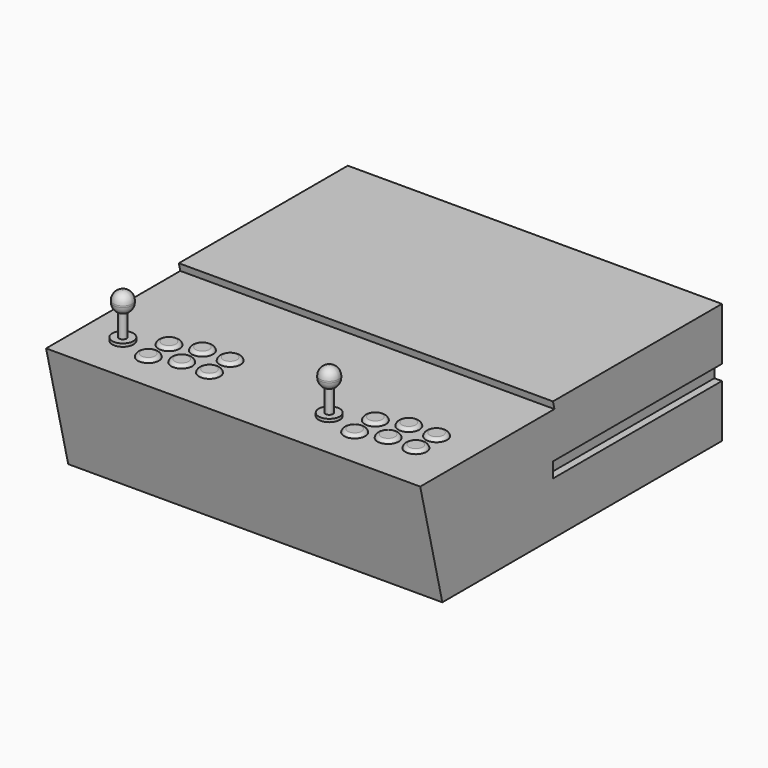
from build123d import *

# Parameters (mm, degrees)
F0_W      = 500
F0_H      = 150
F1_DEPTH  = 500
F3_DEPTH  = 546
F4_W      = 500
F4_H      = 280
F5_DEPTH  = 10
F6_DEPTH  = 2
F7_DEPTH  = 2
F8_W      = 280
F8_H      = 10
F9_DEPTH  = 10
F10_W     = 280
F10_H     = 10
F11_DEPTH = 10
F12_R     = 14
F13_DEPTH = 4
F15_R     = 5
F16_DEPTH = 30
F17_R     = 5
F18_DEPTH = 30
F19_R     = 12.5
F19_R_2   = 5
F20_DEPTH = 25
F22_R     = 12.5
F22_R_2   = 5
F23_DEPTH = 25
F26_DEPTH = 496.001


# Not quite as in the source:
# - a fillet or chamfer that OpenCascade refuses, or shapes differently, is made with other operations: its cross-section is extruded or revolved along the edge and cut away or added


with BuildPart() as f1:
    # F0 (on Front) → F1 (new body)
    with BuildSketch(Plane.XZ):
        with Locations((170.9539443254, 78.5526317079)):
            Rectangle(F0_W, F0_H)
    extrude(amount=F1_DEPTH)

    # F2 (on face) → F3 (cut)
    with BuildSketch(Plane.YZ.offset(420.9539443254)):
        Polygon((-463.3333333489, 3.5526317079), (-500, 153.5526317079), (-500, 3.5526317079), align=None)
    extrude(amount=-F3_DEPTH, mode=Mode.SUBTRACT)

    # F4 (on face) → F5 (join)
    with BuildSketch(Plane.XY.offset(153.5526317079)):
        with Locations((170.9539443254, -140)):
            Rectangle(F4_W, F4_H)
    extrude(amount=F5_DEPTH)

    # F6 (cut): a face of the model
    f6_faces = [f1.faces().sort_by_distance(p)[0] for p in [
        (420.9539443254, -237.1833592457, 82.4533645522),
    ]]
    extrude(f6_faces, amount=-F6_DEPTH, mode=Mode.SUBTRACT)

    # F7 (cut): a face of the model
    f7_faces = [f1.faces().sort_by_distance(p)[0] for p in [
        (-79.0460556746, -237.1833592457, 82.4533645522),
    ]]
    extrude(f7_faces, amount=-F7_DEPTH, mode=Mode.SUBTRACT)

    # F8 (on face) → F9 (cut)
    with BuildSketch(Plane(origin=(-77.0460556746, 0, 0), x_dir=(0, -1, 0), z_dir=(-1, 0, 0))):
        with Locations((140, 88.5526317079)):
            Rectangle(F8_W, F8_H)
        with Locations((140, 78.5526317079)):
            Rectangle(F8_W, F8_H)
    extrude(amount=-F9_DEPTH, mode=Mode.SUBTRACT)

    # F10 (on face) → F11 (cut)
    with BuildSketch(Plane.YZ.offset(418.9539443254)):
        with Locations((-140, 78.5526317079)):
            Rectangle(F10_W, F10_H)
        with Locations((-140, 88.5526317079)):
            Rectangle(F10_W, F10_H)
    extrude(amount=-F11_DEPTH, mode=Mode.SUBTRACT)

    # F12 (on face) → F13 (join)
    with BuildSketch(Plane.XY.offset(153.5526317079)):
        with Locations((-25.8450303767, -436.7535151103)):
            Circle(F12_R)
        with Locations((17.4901243299, -448.7535059452)):
            Circle(F12_R)
        with Locations((52.2069185972, -436.7535114288)):
            Circle(F12_R)
        with Locations((89.009873569, -436.7535151103)):
            Circle(F12_R)
        with Locations((89.009873569, -402.506593571)):
            Circle(F12_R)
        with Locations((52.2069185972, -402.5065898895)):
            Circle(F12_R)
        with Locations((17.4901243299, -414.5065844059)):
            Circle(F12_R)
        with Locations((246.577270329, -435.284647045)):
            Circle(F12_R)
        with Locations((289.9124250357, -447.2846378799)):
            Circle(F12_R)
        with Locations((289.9124250357, -413.0377163406)):
            Circle(F12_R)
        with Locations((324.6292193029, -435.2846433635)):
            Circle(F12_R)
        with Locations((324.6292193029, -401.0377218242)):
            Circle(F12_R)
        with Locations((361.4321742747, -401.0377255057)):
            Circle(F12_R)
        with Locations((361.4321742747, -435.284647045)):
            Circle(F12_R)
    extrude(amount=F13_DEPTH)

    # F14: fillet of radius 5 on 12 edges, made by hand

    # F14_s1 → F14_t2 (revolve, cut)
    with BuildSketch(Plane.XZ.offset(448.7535059452)):
        with BuildLine():
            ThreePointArc((31.4901243299, 153.5526317079), (29.7534225045, 156.4256150541), (26.5911448444, 157.5526317079))
            Line((26.5911448444, 157.5526317079), (31.4901243299, 157.5526317079))
            Line((31.4901243299, 157.5526317079), (31.4901243299, 153.5526317079))
        make_face()
    revolve(axis=Axis((17.4901243299, -448.7535059452, 157.5526317079), (0, 0, 1)), mode=Mode.SUBTRACT)

    # F14_s3 → F14_t4 (revolve, cut)
    with BuildSketch(Plane.XZ.offset(414.5065844059)):
        with BuildLine():
            ThreePointArc((31.4901243299, 153.5526317079), (29.7534225045, 156.4256150541), (26.5911448444, 157.5526317079))
            Line((26.5911448444, 157.5526317079), (31.4901243299, 157.5526317079))
            Line((31.4901243299, 157.5526317079), (31.4901243299, 153.5526317079))
        make_face()
    revolve(axis=Axis((17.4901243299, -414.5065844059, 157.5526317079), (0, 0, 1)), mode=Mode.SUBTRACT)

    # F14_s5 → F14_t6 (revolve, cut)
    with BuildSketch(Plane.XZ.offset(402.5065898895)):
        with BuildLine():
            ThreePointArc((66.2069185972, 153.5526317079), (64.4702167718, 156.4256150541), (61.3079391116, 157.5526317079))
            Line((61.3079391116, 157.5526317079), (66.2069185972, 157.5526317079))
            Line((66.2069185972, 157.5526317079), (66.2069185972, 153.5526317079))
        make_face()
    revolve(axis=Axis((52.2069185972, -402.5065898895, 157.5526317079), (0, 0, 1)), mode=Mode.SUBTRACT)

    # F14_s7 → F14_t8 (revolve, cut)
    with BuildSketch(Plane.XZ.offset(436.7535114288)):
        with BuildLine():
            ThreePointArc((66.2069185972, 153.5526317079), (64.4702167718, 156.4256150541), (61.3079391116, 157.5526317079))
            Line((61.3079391116, 157.5526317079), (66.2069185972, 157.5526317079))
            Line((66.2069185972, 157.5526317079), (66.2069185972, 153.5526317079))
        make_face()
    revolve(axis=Axis((52.2069185972, -436.7535114288, 157.5526317079), (0, 0, 1)), mode=Mode.SUBTRACT)

    # F14_s9 → F14_t10 (revolve, cut)
    with BuildSketch(Plane.XZ.offset(436.7535151103)):
        with BuildLine():
            ThreePointArc((103.009873569, 153.5526317079), (101.2731717436, 156.4256150541), (98.1108940834, 157.5526317079))
            Line((98.1108940834, 157.5526317079), (103.009873569, 157.5526317079))
            Line((103.009873569, 157.5526317079), (103.009873569, 153.5526317079))
        make_face()
    revolve(axis=Axis((89.009873569, -436.7535151103, 157.5526317079), (0, 0, 1)), mode=Mode.SUBTRACT)

    # F14_s11 → F14_t12 (revolve, cut)
    with BuildSketch(Plane.XZ.offset(402.506593571)):
        with BuildLine():
            ThreePointArc((103.009873569, 153.5526317079), (101.2731717436, 156.4256150541), (98.1108940834, 157.5526317079))
            Line((98.1108940834, 157.5526317079), (103.009873569, 157.5526317079))
            Line((103.009873569, 157.5526317079), (103.009873569, 153.5526317079))
        make_face()
    revolve(axis=Axis((89.009873569, -402.506593571, 157.5526317079), (0, 0, 1)), mode=Mode.SUBTRACT)

    # F14_s13 → F14_t14 (revolve, cut)
    with BuildSketch(Plane.XZ.offset(447.2846378799)):
        with BuildLine():
            ThreePointArc((303.9124250356, 153.5526317079), (302.1757232102, 156.4256150541), (299.0134455501, 157.5526317079))
            Line((299.0134455501, 157.5526317079), (303.9124250357, 157.5526317079))
            Line((303.9124250357, 157.5526317079), (303.9124250356, 153.5526317079))
        make_face()
    revolve(axis=Axis((289.9124250357, -447.2846378799, 157.5526317079), (0, 0, 1)), mode=Mode.SUBTRACT)

    # F14_s15 → F14_t16 (revolve, cut)
    with BuildSketch(Plane.XZ.offset(413.0377163406)):
        with BuildLine():
            ThreePointArc((303.9124250356, 153.5526317079), (302.1757232102, 156.4256150541), (299.0134455501, 157.5526317079))
            Line((299.0134455501, 157.5526317079), (303.9124250357, 157.5526317079))
            Line((303.9124250357, 157.5526317079), (303.9124250356, 153.5526317079))
        make_face()
    revolve(axis=Axis((289.9124250357, -413.0377163406, 157.5526317079), (0, 0, 1)), mode=Mode.SUBTRACT)

    # F14_s17 → F14_t18 (revolve, cut)
    with BuildSketch(Plane.XZ.offset(401.0377218242)):
        with BuildLine():
            ThreePointArc((338.6292193029, 153.5526317079), (336.8925174775, 156.4256150541), (333.7302398174, 157.5526317079))
            Line((333.7302398174, 157.5526317079), (338.6292193029, 157.5526317079))
            Line((338.6292193029, 157.5526317079), (338.6292193029, 153.5526317079))
        make_face()
    revolve(axis=Axis((324.6292193029, -401.0377218242, 157.5526317079), (0, 0, 1)), mode=Mode.SUBTRACT)

    # F14_s19 → F14_t20 (revolve, cut)
    with BuildSketch(Plane.XZ.offset(435.2846433635)):
        with BuildLine():
            ThreePointArc((338.6292193029, 153.5526317079), (336.8925174775, 156.4256150541), (333.7302398174, 157.5526317079))
            Line((333.7302398174, 157.5526317079), (338.6292193029, 157.5526317079))
            Line((338.6292193029, 157.5526317079), (338.6292193029, 153.5526317079))
        make_face()
    revolve(axis=Axis((324.6292193029, -435.2846433635, 157.5526317079), (0, 0, 1)), mode=Mode.SUBTRACT)

    # F14_s21 → F14_t22 (revolve, cut)
    with BuildSketch(Plane.XZ.offset(435.284647045)):
        with BuildLine():
            ThreePointArc((375.4321742747, 153.5526317079), (373.6954724493, 156.4256150541), (370.5331947892, 157.5526317079))
            Line((370.5331947892, 157.5526317079), (375.4321742747, 157.5526317079))
            Line((375.4321742747, 157.5526317079), (375.4321742747, 153.5526317079))
        make_face()
    revolve(axis=Axis((361.4321742747, -435.284647045, 157.5526317079), (0, 0, 1)), mode=Mode.SUBTRACT)

    # F14_s23 → F14_t24 (revolve, cut)
    with BuildSketch(Plane.XZ.offset(401.0377255057)):
        with BuildLine():
            ThreePointArc((375.4321742747, 153.5526317079), (373.6954724493, 156.4256150541), (370.5331947892, 157.5526317079))
            Line((370.5331947892, 157.5526317079), (375.4321742747, 157.5526317079))
            Line((375.4321742747, 157.5526317079), (375.4321742747, 153.5526317079))
        make_face()
    revolve(axis=Axis((361.4321742747, -401.0377255057, 157.5526317079), (0, 0, 1)), mode=Mode.SUBTRACT)

    # F15 (on face) → F16 (join)
    with BuildSketch(Plane.XY.offset(157.5526317079)):
        with Locations((-25.8450303767, -436.7535151103)):
            Circle(F15_R)
    extrude(amount=F16_DEPTH)

    # F17 (on face) → F18 (join)
    with BuildSketch(Plane.XY.offset(157.5526317079)):
        with Locations((246.577270329, -435.284647045)):
            Circle(F17_R)
    extrude(amount=F18_DEPTH)

    # F19 (on face) → F20 (join)
    with BuildSketch(Plane.XY.offset(187.5526317079)):
        with Locations((-25.8450303767, -436.7535151103)):
            Circle(F19_R)
        with Locations((-25.8450303767, -436.7535151103)):
            Circle(F19_R_2, mode=Mode.SUBTRACT)
        with Locations((-25.8450303767, -436.7535151103)):
            Circle(F19_R_2)
    extrude(amount=F20_DEPTH)

    # F21: fillet of radius 12 on 2 edges, made by hand

    # F21_s1 → F21_t2 (revolve, cut)
    with BuildSketch(Plane.XZ.offset(436.7535151103)):
        with BuildLine():
            ThreePointArc((-13.3450303767, 200.5526317079), (-16.8597490025, 209.0379130821), (-25.3450303767, 212.5526317079))
            Line((-25.3450303767, 212.5526317079), (-13.3450303767, 212.5526317079))
            Line((-13.3450303767, 212.5526317079), (-13.3450303767, 200.5526317079))
        make_face()
    revolve(axis=Axis((-25.8450303767, -436.7535151103, 212.5526317079), (0, 0, 1)), mode=Mode.SUBTRACT)

    # F21_s3 → F21_t4 (revolve, cut)
    with BuildSketch(Plane.XZ.offset(436.7535151103)):
        with BuildLine():
            ThreePointArc((-13.3450303767, 198.6769294385), (-15.3951560057, 191.968725506), (-20.8450303767, 187.5526317079))
            Line((-20.8450303767, 187.5526317079), (-13.3450303767, 187.5526317079))
            Line((-13.3450303767, 187.5526317079), (-13.3450303767, 198.6769294385))
        make_face()
    revolve(axis=Axis((-25.8450303767, -436.7535151103, 187.5526317079), (0, 0, 1)), mode=Mode.SUBTRACT)

    # F22 (on face) → F23 (join)
    with BuildSketch(Plane.XY.offset(187.5526317079)):
        with Locations((246.577270329, -435.284647045)):
            Circle(F22_R)
        with Locations((246.577270329, -435.284647045)):
            Circle(F22_R_2, mode=Mode.SUBTRACT)
        with Locations((246.577270329, -435.284647045)):
            Circle(F22_R_2)
    extrude(amount=F23_DEPTH)

    # F24: fillet of radius 12 on 2 edges, made by hand

    # F24_s1 → F24_t2 (revolve, cut)
    with BuildSketch(Plane.XZ.offset(435.284647045)):
        with BuildLine():
            ThreePointArc((259.077270329, 200.5526317079), (255.5625517032, 209.0379130821), (247.077270329, 212.5526317079))
            Line((247.077270329, 212.5526317079), (259.077270329, 212.5526317079))
            Line((259.077270329, 212.5526317079), (259.077270329, 200.5526317079))
        make_face()
    revolve(axis=Axis((246.577270329, -435.284647045, 212.5526317079), (0, 0, 1)), mode=Mode.SUBTRACT)

    # F24_s3 → F24_t4 (revolve, cut)
    with BuildSketch(Plane.XZ.offset(435.284647045)):
        with BuildLine():
            ThreePointArc((259.077270329, 198.6769294385), (257.0271447001, 191.968725506), (251.577270329, 187.5526317079))
            Line((251.577270329, 187.5526317079), (259.077270329, 187.5526317079))
            Line((259.077270329, 187.5526317079), (259.077270329, 198.6769294385))
        make_face()
    revolve(axis=Axis((246.577270329, -435.284647045, 187.5526317079), (0, 0, 1)), mode=Mode.SUBTRACT)

    # F25 (on face) → F26 (cut, through all)
    with BuildSketch(Plane.YZ.offset(418.9539443254)):
        Polygon((-277.5555555566, 153.5526317079), (-280, 163.5526317079), (-280, 153.5526317079), align=None)
    extrude(amount=-F26_DEPTH, mode=Mode.SUBTRACT)


solid = f1.part
